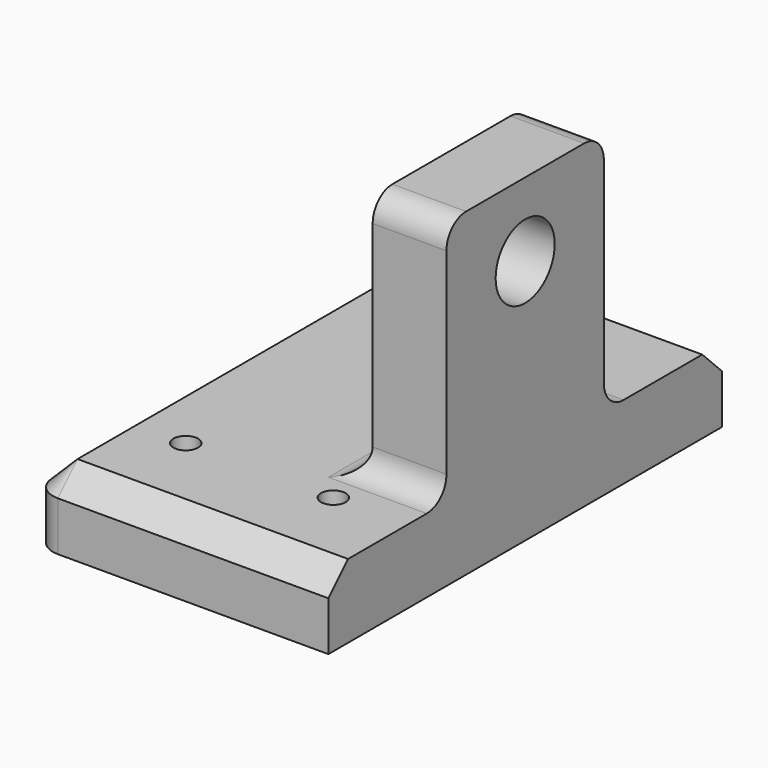
from build123d import *

# Parameters (mm, degrees)
F1_DEPTH = 15
F2_W     = 40
F2_H     = 50
F3_DEPTH = 15
F4_R     = 5
F5_SIZE  = 4.99999
F6_R     = 7.5
F7_DEPTH = 25
F8_R     = 2.5
F9_DEPTH = 25


# Not quite as in the source:
# - a fillet or chamfer is up to 0.001 mm smaller than in the source, because OpenCascade refuses the exact size


with BuildPart() as f1:
    # F0 (on Top) → F1 (new body)
    with BuildSketch(Plane.XY):
        with BuildLine():
            Line((-5.0826547947, 51.5897747652), (-60.0826547947, 51.5897747652))
            ThreePointArc((-60.0826547947, 51.5897747652), (-63.6181887006, 50.1253086711), (-65.0826547947, 46.5897747652))
            Line((-65.0826547947, 46.5897747652), (-65.0826547947, -43.4102252348))
            ThreePointArc((-65.0826547947, -43.4102252348), (-63.6181887006, -46.9457591408), (-60.0826547947, -48.4102252348))
            Line((-60.0826547947, -48.4102252348), (-5.0826547947, -48.4102252348))
            Line((-5.0826547947, -48.4102252348), (-5.0826547947, 51.5897747652))
        make_face()
    extrude(amount=F1_DEPTH)

    # F2 (on face) → F3 (join)
    with BuildSketch(Plane.YZ.offset(-5.0826547947)):
        with Locations((1.5897747652, 40)):
            Rectangle(F2_W, F2_H)
    extrude(amount=-F3_DEPTH)

    # F4
    f4_edges = [f1.edges().sort_by_distance(p)[0] for p in [
        (-12.582655, 21.589775, 65),
        (-12.582655, -18.410225, 65),
        (-12.582655, -18.410225, 15),
        (-20.082655, 1.589775, 15),
        (-12.582655, 21.589775, 15),
    ]]
    fillet(f4_edges, radius=F4_R)

    # F5 (size 5 in the source; OpenCascade refuses exactly that, so slightly less here)
    f5_edges = [f1.edges().sort_by_distance(p)[0] for p in [
        (-32.582655, 51.589775, 15),
    ]]
    chamfer(f5_edges, length=F5_SIZE)

    # F6 (on face) → F7 (cut)
    with BuildSketch(Plane(origin=(-20.0826547947, 0, 0), x_dir=(0, -1, 0), z_dir=(-1, 0, 0))):
        with Locations((-1.5897747652, 50)):
            Circle(F6_R)
    extrude(amount=-F7_DEPTH, mode=Mode.SUBTRACT)

    # F8 (on face) → F9 (cut)
    with BuildSketch(Plane(origin=(0, 0, 0), x_dir=(1, 0, 0), z_dir=(0, 0, -1))):
        with Locations((-20.0826547947, -31.5897747652)):
            Circle(F8_R)
        with Locations((-50.0826547947, -31.5897747652)):
            Circle(F8_R)
        with Locations((-50.0826547947, 28.4102252348)):
            Circle(F8_R)
        with Locations((-20.0826547947, 28.4102252348)):
            Circle(F8_R)
    extrude(amount=-F9_DEPTH, mode=Mode.SUBTRACT)


solid = f1.part
